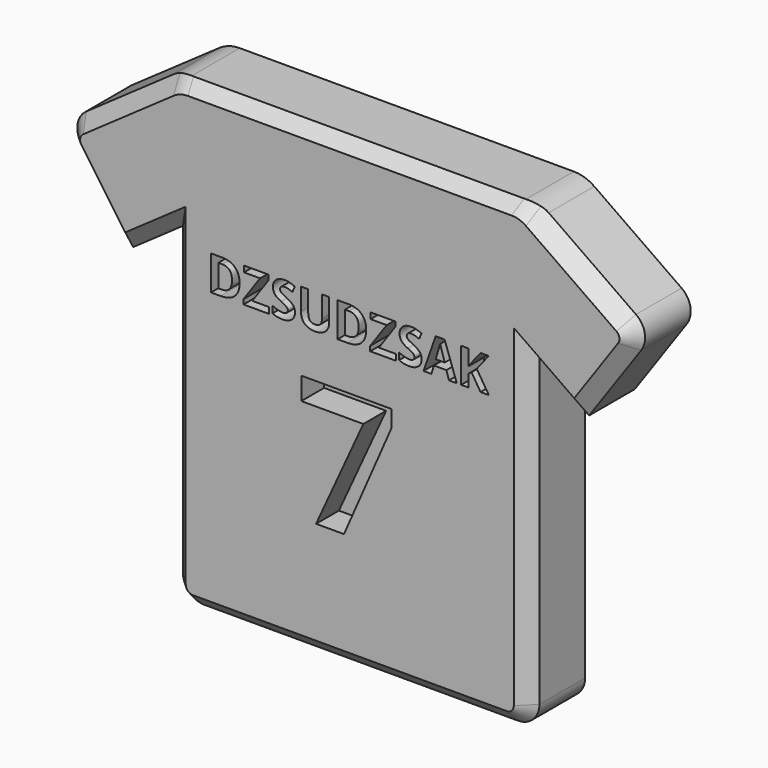
from build123d import *

# Parameters (mm, degrees)
F1_DEPTH       = 10
F2_TEXT_SIZE   = 6.762289669
F2_TEXT_SIZE_2 = 24.7082084469
F3_DEPTH       = 4
F4_R           = 3
F5_SIZE        = 2
F6_SIZE        = 2
F7_SIZE        = 1.6
F8_SIZE        = 2
F9_R           = 5
F10_R          = 5


# Not quite as in the source:
# - a feature names something its author has since deleted; it is built from what else it names
# - Text() gives the source's letters only with a copy of the font that has no kerning and outlines rounded to 1/6400 em; it was checked with that copy


with BuildPart() as f1:
    # F0 (on Front) → F1 (new body)
    with BuildSketch(Plane.XZ):
        Polygon((25, 17.1502526636), (25, 36.3584065651), (15.9751197599, 23.4695418392), align=None)
        Polygon((40.9902705448, 25.1618985917), (25, 36.3584065651), (25, 17.1502526636), (31.9653903047, 12.2730338657), align=None)
        with BuildLine():
            Line((25, 36.3584065651), (0, 36.3584065651))
            Line((0, 36.3584065651), (0, -28.6415934349))
            Line((0, -28.6415934349), (22, -28.6415934349))
            ThreePointArc((22, -28.6415934349), (24.1213203436, -27.7629137784), (25, -25.6415934349))
            Line((25, -25.6415934349), (25, 17.1502526636))
            Line((25, 17.1502526636), (15.9751197599, 23.4695418392))
            Line((15.9751197599, 23.4695418392), (25, 36.3584065651))
        make_face()
        Polygon((-25, 17.1502526636), (-25, 36.3584065651), (-40.9902705448, 25.1618985917), (-31.9653903047, 12.2730338657), align=None)
        with BuildLine():
            Line((0, -28.6415934349), (0, 36.3584065651))
            Line((0, 36.3584065651), (-25, 36.3584065651))
            Line((-25, 36.3584065651), (-24.9732798206, 36.3202461942))
            Line((-24.9732798206, 36.3202461942), (-15.9751197599, 23.4695418392))
            Line((-15.9751197599, 23.4695418392), (-25, 17.1502526636))
            Line((-25, 17.1502526636), (-25, -25.6415934349))
            ThreePointArc((-25, -25.6415934349), (-24.1213203436, -27.7629137784), (-22, -28.6415934349))
            Line((-22, -28.6415934349), (0, -28.6415934349))
        make_face()
        with BuildLine():
            Line((25, 36.3584065651), (0, 36.3584065651))
            Line((0, 36.3584065651), (0, -28.6415934349))
            Line((0, -28.6415934349), (22, -28.6415934349))
            ThreePointArc((22, -28.6415934349), (24.1213203436, -27.7629137784), (25, -25.6415934349))
            Line((25, -25.6415934349), (25, 17.1502526636))
            Line((25, 17.1502526636), (15.9751197599, 23.4695418392))
            Line((15.9751197599, 23.4695418392), (25, 36.3584065651))
        make_face()
        Polygon((-24.9732798206, 36.3202461942), (-25, 36.3584065651), (-25, 17.1502526636), (-15.9751197599, 23.4695418392), align=None)
    extrude(amount=F1_DEPTH)

    # F2 (on face) → F3 (cut)
    with BuildSketch(Plane.XZ.offset(10)):
        with Locations((-20.0628023595, 11.5509793764)):
            Text('DZSUDZSAK', F2_TEXT_SIZE, font='Open Sans', font_style=FontStyle.BOLD, text_align=(TextAlign.LEFT, TextAlign.BOTTOM))
        with Locations((-7.4607207537, -12.2157381848)):
            Text('7', F2_TEXT_SIZE_2, font='Open Sans', font_style=FontStyle.BOLD, text_align=(TextAlign.LEFT, TextAlign.BOTTOM))
    extrude(amount=-F3_DEPTH, mode=Mode.SUBTRACT)

    # F4
    f4_edges = [f1.edges().sort_by_distance(p)[0] for p in [
        (-40.990271, -5, 25.161899),
        (40.990271, -5, 25.161899),
    ]]
    fillet(f4_edges, radius=F4_R)

    # F5
    f5_edges = [f1.edges().sort_by_distance(p)[0] for p in [
        (-31.766407, -10, 31.620517),
    ]]
    chamfer(f5_edges, length=F5_SIZE)

    # F6
    f6_edges = [f1.edges().sort_by_distance(p)[0] for p in [
        (31.766407, -10, 31.620517),
        (35.617466, -10, 17.488738),
    ]]
    chamfer(f6_edges, length=F6_SIZE)

    # F7
    f7_edges = [f1.edges().sort_by_distance(p)[0] for p in [
        (0, -10, 36.358407),
    ]]
    chamfer(f7_edges, length=F7_SIZE)

    # F8
    f8_edges = [f1.edges().sort_by_distance(p)[0] for p in [
        (27.663543, -10, 15.28522),
        (25, -10, -4.24567),
        (-27.663543, -10, 15.28522),
    ]]
    chamfer(f8_edges, length=F8_SIZE)

    # F9 (call 1 of 2: OpenCascade refuses the feature's edges together)
    f9_edges = [f1.edges().sort_by_distance(p)[0] for p in [
        (-25, -4, 36.358407),
    ]]
    fillet(f9_edges, radius=F9_R)

    # F9#2 (call 2 of 2)
    f9_2_edges = [f1.edges().sort_by_distance(p)[0] for p in [
        (-24.050382, -9.2, 35.558407),
    ]]
    fillet(f9_2_edges, radius=F9_R)

    # F10 (call 1 of 2: OpenCascade refuses the feature's edges together)
    f10_edges = [f1.edges().sort_by_distance(p)[0] for p in [
        (25, -4, 36.358407),
    ]]
    fillet(f10_edges, radius=F10_R)

    # F10#2 (call 2 of 2)
    f10_2_edges = [f1.edges().sort_by_distance(p)[0] for p in [
        (24.050382, -9.2, 35.558407),
    ]]
    fillet(f10_2_edges, radius=F10_R)


solid = f1.part
